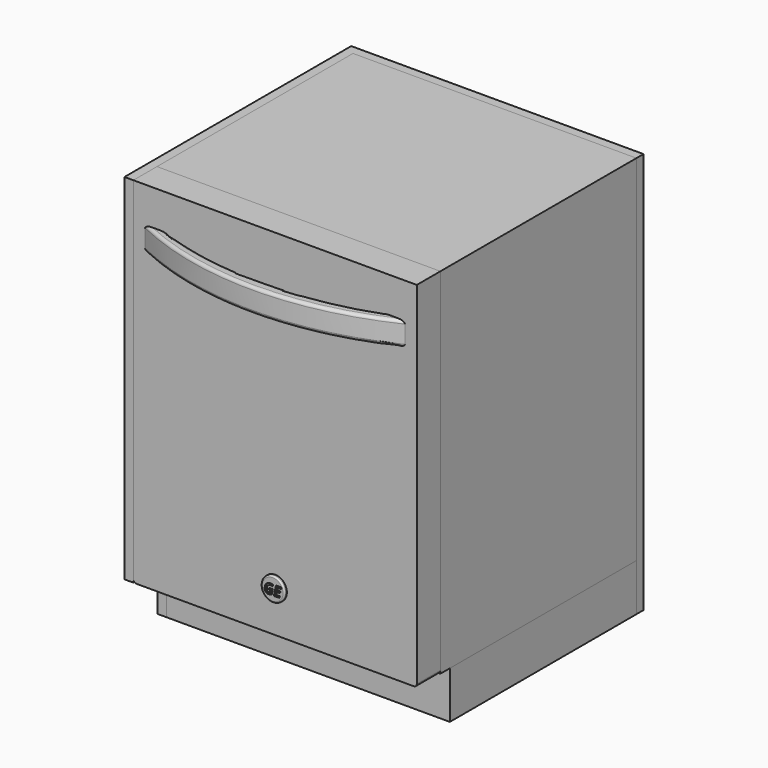
from build123d import *

# Parameters (mm, degrees)
F0_W          = 609.6
F0_H          = 762
F0_R          = 25.4
F0_W_2        = 558.8
F0_H_2        = 50.8
F1_DEPTH      = 63.5
F0_H_3        = 101.6
F2_DEPTH      = 527.05
F3_DEPTH      = 127
F4_W          = 457.2
F4_H          = 38.1
F5_DEPTH      = 787.401
F6_T1_DEPTH   = 50.8
F6_T3_DEPTH   = 50.8
F6_T5_DEPTH   = 1447.8
F6_T7_DEPTH   = 1447.8
F7_R          = 6.35
F8_DEPTH      = 527.05
F9_R          = 6.35
F10_DEPTH     = 69.85
F11_R         = 3.175
F12_TEXT_SIZE = 30.0888450148
F13_DEPTH     = 3.175
F14_DEPTH     = 25.4
F15_W         = 609.6
F15_H         = 863.6
F16_DEPTH     = 19.05
F18_DEPTH     = 19.05


# Not quite as in the source:
# - a fillet or chamfer that OpenCascade refuses, or shapes differently, is made with other operations: its cross-section is extruded or revolved along the edge and cut away or added
# - Text() gives the source's letters only with a copy of the font that has no kerning and outlines rounded to 1/6400 em; it was checked with that copy


with BuildPart() as f1:
    # F0 (on Front) → F1 (new body)
    with BuildSketch(Plane.XZ):
        with Locations((0, 50.8)):
            Rectangle(F0_W, F0_H)
        with Locations((0, -241.3)):
            Circle(F0_R, mode=Mode.SUBTRACT)
        with Locations((0, 330.2)):
            Rectangle(F0_W_2, F0_H_2, mode=Mode.SUBTRACT)
        with Locations((0, 330.2)):
            Rectangle(F0_W_2, F0_H_2)
        with Locations((0, -241.3)):
            Circle(F0_R)
    extrude(amount=F1_DEPTH)

    # F0 (on Front) → F3 (join)
    with BuildSketch(Plane.XZ):
        with Locations((0, 330.2)):
            Rectangle(F0_W_2, F0_H_2)
    extrude(amount=F3_DEPTH)

    # F4 (on face) → F5 (cut, through all)
    with BuildSketch(Plane.XY.offset(355.6)):
        with Locations((0, -82.55)):
            Rectangle(F4_W, F4_H)
    extrude(amount=-F5_DEPTH, mode=Mode.SUBTRACT)

    # F6: fillet of radius 646.43 on 4 edges, made by hand

    # F6_s2 → F6_t1 (join)
    with BuildSketch(Plane.XY.offset(304.8)):
        with BuildLine():
            ThreePointArc((-228.6, -63.5), (-120.9240321185, -92.0037721886), (-9.9533535588, -101.6))
            Line((-9.9533535588, -101.6), (-9.9533535588, -114.5286))
            Line((-9.9533535588, -114.5286), (-228.6, -114.5286))
            Line((-228.6, -114.5286), (-241.5286, -101.6))
            ThreePointArc((-241.5286, -101.6), (-241.5286, -82.55), (-232.9729329288, -75.6666))
            Line((-232.9729329288, -75.6666), (-228.6, -63.5))
        make_face()
    extrude(amount=F6_T1_DEPTH)

    # F6_s4 → F6_t3 (join)
    with BuildSketch(Plane.XY.offset(304.8)):
        with BuildLine():
            ThreePointArc((228.6, -63.5), (120.9240321185, -92.0037721886), (9.9533535588, -101.6))
            Line((9.9533535588, -101.6), (9.9533535588, -114.5286))
            Line((9.9533535588, -114.5286), (228.6, -114.5286))
            Line((228.6, -114.5286), (241.5286, -101.6))
            ThreePointArc((241.5286, -101.6), (241.5286, -82.55), (232.9729329288, -75.6666))
            Line((232.9729329288, -75.6666), (228.6, -63.5))
        make_face()
    extrude(amount=F6_T3_DEPTH)

    # F6_s6 → F6_t5 (cut)
    with BuildSketch(Plane.XY.offset(-393.7)):
        with BuildLine():
            ThreePointArc((-279.4, -63.5), (-143.262529993, -110.9251319693), (0, -127))
            Line((0, -127), (0, -139.9286))
            Line((0, -139.9286), (-279.4, -139.9286))
            Line((-279.4, -139.9286), (-292.3286, -127))
            ThreePointArc((-292.3286, -127), (-292.3286, -95.25), (-284.988, -75.1586))
            Line((-284.988, -75.1586), (-279.4, -63.5))
        make_face()
    extrude(amount=F6_T5_DEPTH, mode=Mode.SUBTRACT)

    # F6_s8 → F6_t7 (cut)
    with BuildSketch(Plane.XY.offset(-393.7)):
        with BuildLine():
            ThreePointArc((279.4, -63.5), (143.262529993, -110.9251319693), (0, -127))
            Line((0, -127), (0, -139.9286))
            Line((0, -139.9286), (279.4, -139.9286))
            Line((279.4, -139.9286), (292.3286, -127))
            ThreePointArc((292.3286, -127), (292.3286, -95.25), (284.988, -75.1586))
            Line((284.988, -75.1586), (279.4, -63.5))
        make_face()
    extrude(amount=F6_T7_DEPTH, mode=Mode.SUBTRACT)

    # F7
    f7_edges = [f1.edges().sort_by_distance(p)[0] for p in [
        (0, -127, 355.6),
        (0, -101.6, 355.6),
        (0, -127, 304.8),
        (0, -101.6, 304.8),
    ]]
    fillet(f7_edges, radius=F7_R)


with BuildPart() as f2:
    # F0 (on Front) → F2 (new body)
    with BuildSketch(Plane.XZ):
        with Locations((0, -381)):
            Rectangle(F0_W, F0_H_3)
    extrude(amount=-F2_DEPTH)

    # F14 (cut): a face of the model
    f14_faces = [f2.faces().sort_by_distance(p)[0] for p in [
        (0, 0, -381),
    ]]
    extrude(f14_faces, amount=-F14_DEPTH, mode=Mode.SUBTRACT)


with BuildPart() as f8:
    # F8 (new, through all): a face of the model
    f8_faces = [f1.part.faces().sort_by_distance(p)[0] for p in [
        (0, 0, 50.8),
    ]]
    extrude(f8_faces, amount=F8_DEPTH)


with BuildPart() as f1_1:
    add(f1.part)

    # F9
    f9_edges = [f1_1.edges().sort_by_distance(p)[0] for p in [
        (-304.8, -31.75, -330.2),
        (304.8, -31.75, -330.2),
    ]]
    fillet(f9_edges, radius=F9_R)


with BuildPart() as f10:
    # F0 (on Front) → F10 (new body)
    with BuildSketch(Plane.XZ):
        with Locations((0, -241.3)):
            Circle(F0_R)
    extrude(amount=F10_DEPTH)

    # F11
    f11_edges = [f10.edges().sort_by_distance(p)[0] for p in [
        (-25.4, -69.85, -241.3),
    ]]
    fillet(f11_edges, radius=F11_R)

    # F12 (on face) → F13 (cut)
    with BuildSketch(Plane.XZ.offset(69.85)):
        with Locations((-19.1044491183, -252.8377498543)):
            Text('GE', F12_TEXT_SIZE, font='Open Sans', font_style=FontStyle.BOLDITALIC, text_align=(TextAlign.LEFT, TextAlign.BOTTOM))
    extrude(amount=-F13_DEPTH, mode=Mode.SUBTRACT)


with BuildPart() as f16:
    # F15 (on face) → F16 (new body)
    with BuildSketch(Plane(origin=(0, 527.05, 0), x_dir=(-1, 0, 0), z_dir=(0, 1, 0))):
        Rectangle(F15_W, F15_H)
    extrude(amount=F16_DEPTH)

    # F17 (on face) → F18 (join)
    with BuildSketch(Plane(origin=(-304.8, 0, 0), x_dir=(0, -1, 0), z_dir=(-1, 0, 0))):
        Polygon((63.5, 431.8), (-546.1, 431.8), (-546.1, -431.8), (-25.4, -431.8), (-25.4, -330.2), (63.5, -330.2), align=None)
    extrude(amount=F18_DEPTH)


solid = Compound([f2.part, f8.part, f1_1.part, f10.part, f16.part])
